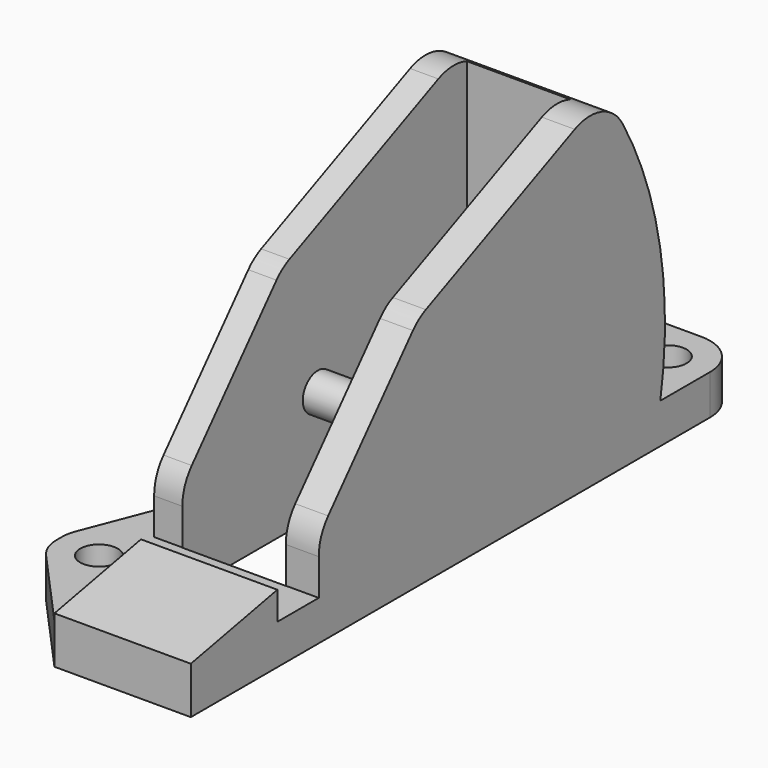
from build123d import *

# Parameters (mm, degrees)
F0_R         = 4
F1_DEPTH     = 8.5
F2_R         = 8
F4_DEPTH     = 29
F5_R         = 4
F6_DEPTH     = 35
F7_W         = 22
F7_H         = 75.6632985204
F8_DEPTH     = 72.001
F9_DEPTH     = 35
F10_T1_DEPTH = 80.2241965153
F10_T3_DEPTH = 17.8781354595
F10_T5_DEPTH = 16.8781354595
F10_T7_DEPTH = 25.8982236505
F10_T9_DEPTH = 24.8982236505


# Not quite as in the source:
# - a fillet or chamfer that OpenCascade refuses, or shapes differently, is made with other operations: its cross-section is extruded or revolved along the edge and cut away or added


with BuildPart() as f1:
    # F0 (on Top) → F1 (new body)
    with BuildSketch(Plane.XY):
        with BuildLine():
            Line((0, 68), (0, 0))
            Line((0, 0), (35, 0))
            Line((35, 0), (35, 68))
            Line((35, 68), (35, 81))
            ThreePointArc((35, 81), (32.3639610307, 87.3639610307), (26, 90))
            Line((26, 90), (12, 90))
            Line((12, 90), (0, 68))
        make_face()
        with Locations((26, 81)):
            Circle(F0_R, mode=Mode.SUBTRACT)
        Polygon((35, 0), (0, 0), (-12, -31), (-12, -37), (6, -57), (35, -57), align=None)
        with Locations((-3, -33.8997244835)):
            Circle(F0_R, mode=Mode.SUBTRACT)
    extrude(amount=F1_DEPTH)

    # F2
    f2_edges = [f1.edges().sort_by_distance(p)[0] for p in [
        (-12, -37, 4.25),
        (-12, -31, 4.25),
    ]]
    fillet(f2_edges, radius=F2_R)

    # F3 (on face) → F4 (join, through all)
    with BuildSketch(Plane.YZ.offset(35)):
        Polygon((-57, 10), (-57, 0), (-34, 0), (-34, 14.5), align=None)
    extrude(amount=-F4_DEPTH)

    # F5 (on face) → F6 (join, through all)
    with BuildSketch(Plane.YZ.offset(35)):
        with BuildLine():
            Line((-23, 20), (-23, 8.5))
            Line((-23, 8.5), (67.7691474557, 8.5))
            ThreePointArc((67.7691474557, 8.5), (66.7805333738, 41.7873112781), (52.7728251344, 72))
            Line((52.7728251344, 72), (3.4575131106, 50))
            Line((3.4575131106, 50), (-23, 20))
        make_face()
        with Locations((13, 23)):
            Circle(F5_R, mode=Mode.SUBTRACT)
    extrude(amount=-F6_DEPTH)

    # F7 (on Top) → F8 (cut, through all)
    with BuildSketch(Plane.XY):
        with Locations((17, 14.7745097056)):
            Rectangle(F7_W, F7_H)
    extrude(amount=F8_DEPTH, mode=Mode.SUBTRACT)

    # F5 (on face) → F9 (join, through all)
    with BuildSketch(Plane.YZ.offset(35)):
        with Locations((13, 23)):
            Circle(F5_R)
    extrude(amount=-F9_DEPTH)

    # F10: fillet of radius 10 on 5 edges, made by hand

    # F10_s2 → F10_t1 (cut)
    with BuildSketch(Plane.YZ.offset(-22.6120982577)):
        with BuildLine():
            ThreePointArc((57.7430836083, 64.4431720463), (52.1704386948, 68.9292292294), (45.0268385832, 68.5444463974))
            Line((45.0268385832, 68.5444463974), (52.7728251344, 72))
            ThreePointArc((52.7728251344, 72), (55.3610878115, 68.2894186982), (57.7430836083, 64.4431720463))
        make_face()
    extrude(amount=F10_T1_DEPTH, mode=Mode.SUBTRACT)

    # F10_s4 → F10_t3 (cut)
    with BuildSketch(Plane.YZ.offset(22.5609322702)):
        with BuildLine():
            ThreePointArc((5.4443969789, 50.886366593), (3.5960570103, 49.8115072456), (2.0184710529, 48.3682796811))
            Line((2.0184710529, 48.3682796811), (3.4575131106, 50))
            Line((3.4575131106, 50), (5.4443969789, 50.886366593))
        make_face()
    extrude(amount=F10_T3_DEPTH, mode=Mode.SUBTRACT)

    # F10_s6 → F10_t5 (cut)
    with BuildSketch(Plane.YZ.offset(-5.4390677298)):
        with BuildLine():
            ThreePointArc((5.4443969789, 50.886366593), (3.5960570103, 49.8115072456), (2.0184710529, 48.3682796811))
            Line((2.0184710529, 48.3682796811), (3.4575131106, 50))
            Line((3.4575131106, 50), (5.4443969789, 50.886366593))
        make_face()
    extrude(amount=F10_T5_DEPTH, mode=Mode.SUBTRACT)

    # F10_s8 → F10_t7 (cut)
    with BuildSketch(Plane.YZ.offset(18.5508881748)):
        with BuildLine():
            ThreePointArc((-23, 16.2203552699), (-22.3541434669, 19.7558891758), (-20.5, 22.8347335476))
            Line((-20.5, 22.8347335476), (-23, 20))
            Line((-23, 20), (-23, 16.2203552699))
        make_face()
    extrude(amount=F10_T7_DEPTH, mode=Mode.SUBTRACT)

    # F10_s10 → F10_t9 (cut)
    with BuildSketch(Plane.YZ.offset(-9.4491118252)):
        with BuildLine():
            ThreePointArc((-20.5, 22.8347335476), (-22.3541434669, 19.7558891758), (-23, 16.2203552699))
            Line((-23, 16.2203552699), (-23, 20))
            Line((-23, 20), (-20.5, 22.8347335476))
        make_face()
    extrude(amount=F10_T9_DEPTH, mode=Mode.SUBTRACT)


solid = f1.part
